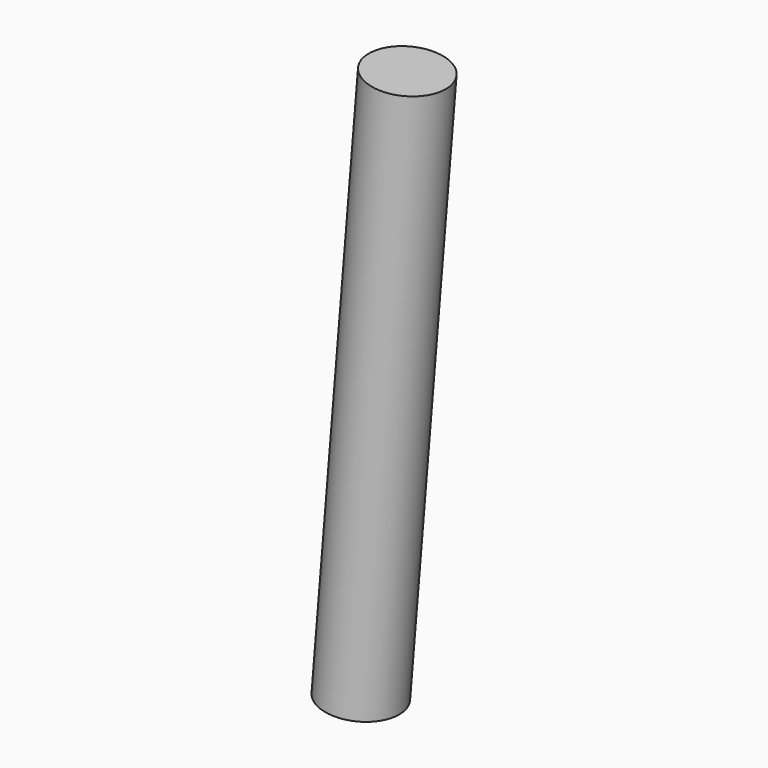
from build123d import *

# Parameters (mm, degrees)
F2_R = 50.8


with BuildPart() as f3:
    # F3: sweep along a path in F0
    with BuildLine(Plane.XZ) as f3_path:
        Line((213.8027258659, -138.2331094519), (152.6, -882.7))
    # F2 (on face) → F3 (sweep)
    with BuildSketch(Plane(origin=(-40.453949994, 0, -492.0798205685), x_dir=(0.9966377797, 0, -0.0819337295), z_dir=(-0.0819337295, 0, -0.9966377797))):
        with Locations((224.4098282015, 0)):
            Circle(F2_R)
    sweep(path=f3_path.line)


solid = f3.part
